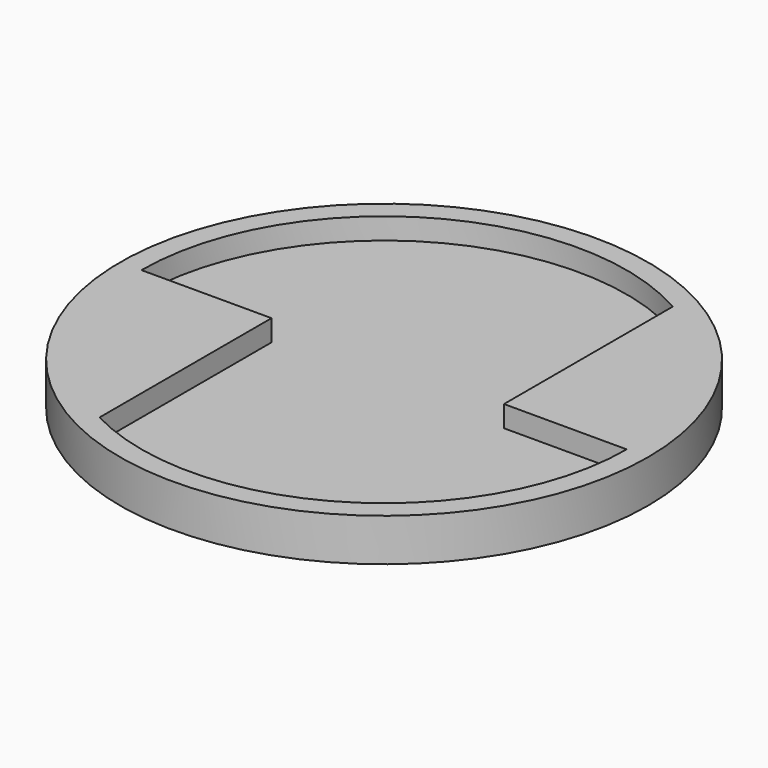
from build123d import *

# Parameters (mm, degrees)
F0_R     = 31.4391719437
F1_DEPTH = 5.08
F2_T     = -2.54
F4_DEPTH = 2.54


# Not quite as in the source:
# - a feature names something its author has since deleted; it is built from what else it names


with BuildPart() as f1:
    # F0 (on Top) → F1 (new body)
    with BuildSketch(Plane.XY):
        Circle(F0_R)
    extrude(amount=F1_DEPTH)

    # F2
    f2_openings = [f1.faces().sort_by_distance(p)[0] for p in [
        (0, 0, 5.08),
    ]]
    offset(amount=F2_T, openings=f2_openings)

    # F3 (on face) → F4 (join)
    with BuildSketch(Plane.XY.offset(2.54)):
        with BuildLine():
            Line((-13.4078683332, 0), (-28.8991719437, 0))
            ThreePointArc((-28.8991719437, 0), (-24.7248703878, -14.9613810638), (-13.4078683332, -25.6006094808))
            Line((-13.4078683332, -25.6006094808), (-13.4078683332, 0))
        make_face()
        with BuildLine():
            ThreePointArc((28.8991719437, 0), (24.9790772251, 14.5329914336), (14.2822936177, 25.1232606969))
            Line((14.2822936177, 25.1232606969), (14.2822936177, 0))
            Line((14.2822936177, 0), (28.8991719437, 0))
        make_face()
    extrude(amount=F4_DEPTH)


solid = f1.part
